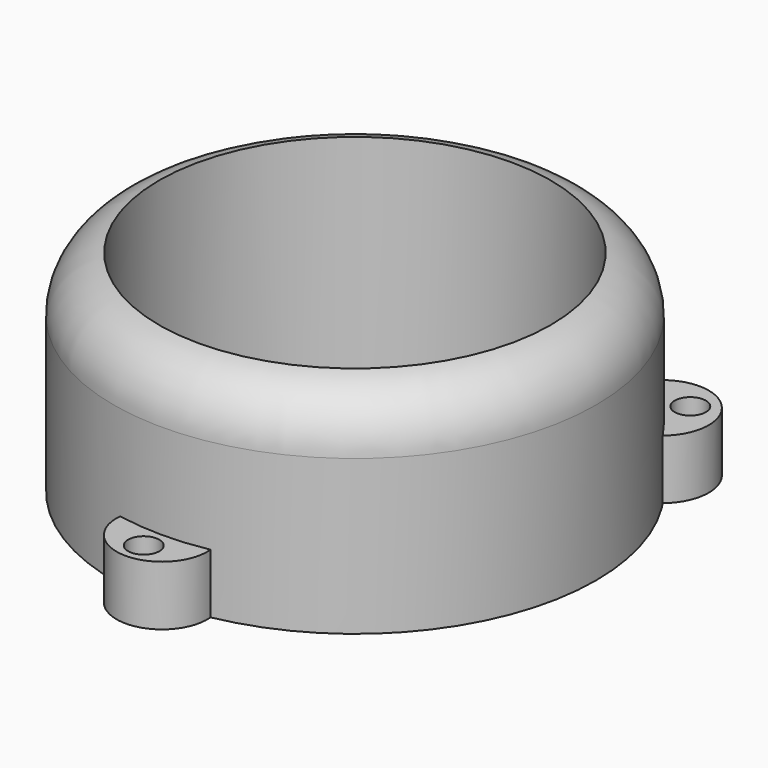
from build123d import *

# Parameters (mm, degrees)
F0_R     = 21.59
F0_R_2   = 17.526
F1_DEPTH = 18.796
F2_R     = 1.397
F3_DEPTH = 5.334
F5_DEPTH = 5.32335


# Not quite as in the source:
# - a fillet or chamfer that OpenCascade refuses, or shapes differently, is made with other operations: its cross-section is extruded or revolved along the edge and cut away or added


with BuildPart() as f1:
    # F0 (on Top) → F1 (new body)
    with BuildSketch(Plane.XY):
        Circle(F0_R)
        Circle(F0_R_2, mode=Mode.SUBTRACT)
    extrude(amount=F1_DEPTH)

    # F2 (on face) → F3 (join)
    with BuildSketch(Plane(origin=(0, 0, 0), x_dir=(1, 0, 0), z_dir=(0, 0, -1))):
        with BuildLine():
            ThreePointArc((-21.2075058824, -4.0459602383), (-21.5081828799, 0), (-21.2075058824, 4.0459602383))
            ThreePointArc((-21.2075058824, 4.0459602383), (-25.5653001948, 0), (-21.2075058824, -4.0459602383))
        make_face()
        with Locations((-23.622, 0)):
            Circle(F2_R, mode=Mode.SUBTRACT)
        with BuildLine():
            ThreePointArc((-4.0459602383, 21.2075058824), (0, 21.59), (4.0459602383, 21.2075058824))
            ThreePointArc((4.0459602383, 21.2075058824), (0, 25.6437689885), (-4.0459602383, 21.2075058824))
        make_face()
        with Locations((0, 23.622)):
            Circle(F2_R, mode=Mode.SUBTRACT)
    extrude(amount=-F3_DEPTH)

    # F4 (on face) → F5 (join)
    with BuildSketch(Plane.XY.offset(5.334)):
        with BuildLine():
            ThreePointArc((15.2619734187, 15.2619734187), (16.6668392005, 13.6913700024), (17.9108306766, 11.990508996))
            ThreePointArc((17.9108306766, 11.990508996), (19.4564957211, 15.0391701429), (18.2294215901, 18.2294215901))
            Line((18.2294215901, 18.2294215901), (17.6633479303, 17.6633479303))
            ThreePointArc((17.6633479303, 17.6633479303), (17.9661794639, 17.210128512), (18.072519757, 16.675519757))
            ThreePointArc((18.072519757, 16.675519757), (17.210128512, 15.3848600501), (15.6876915837, 15.6876915837))
            Line((15.6876915837, 15.6876915837), (15.2619734187, 15.2619734187))
        make_face()
        with BuildLine():
            Line((17.6633479303, 17.6633479303), (18.2294215901, 18.2294215901))
            ThreePointArc((18.2294215901, 18.2294215901), (15.0665422687, 19.4578041419), (12.025389791, 17.9531045364))
            ThreePointArc((12.025389791, 17.9531045364), (13.7098474372, 16.6871156464), (15.2619734187, 15.2619734187))
            Line((15.2619734187, 15.2619734187), (15.6876915837, 15.6876915837))
            ThreePointArc((15.6876915837, 15.6876915837), (15.6876915837, 17.6633479303), (17.6633479303, 17.6633479303))
        make_face()
    extrude(amount=-F5_DEPTH)

    # F6: fillet of radius 5.08 on 1 edges, made by hand

    # F6_s1 → F6_t2 (revolve, cut)
    with BuildSketch(Plane.XZ):
        with BuildLine():
            ThreePointArc((21.59, 13.8186368427), (20.4449510797, 17.0315109454), (17.526, 18.796))
            Line((17.526, 18.796), (21.59, 18.796))
            Line((21.59, 18.796), (21.59, 13.8186368427))
        make_face()
    revolve(axis=Axis((0, 0, 18.796), (0, 0, 1)), mode=Mode.SUBTRACT)


solid = f1.part
